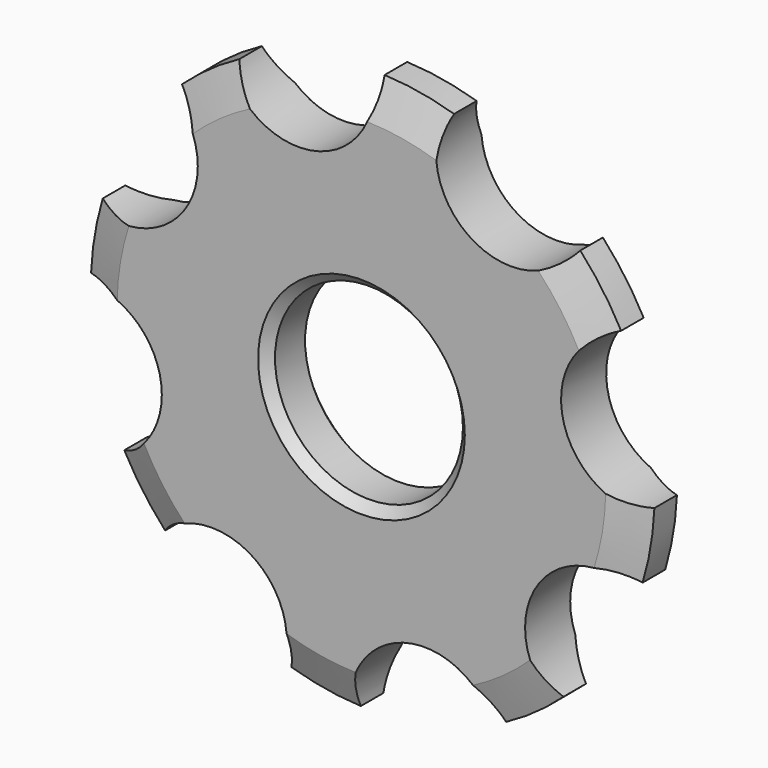
from build123d import *

# Parameters (mm, degrees)
F0_R         = 5
F1_DEPTH     = 3
F2_C1_SIZE2  = 0.75
F2_C1_SIZE   = 2
F2_C2_SIZE2  = 0.75
F2_C2_SIZE   = 2
F2_C3_SIZE2  = 0.75
F2_C3_SIZE   = 2
F2_C4_SIZE2  = 0.75
F2_C4_SIZE   = 2
F2_C5_SIZE2  = 0.75
F2_C5_SIZE   = 2
F2_C6_SIZE2  = 0.75
F2_C6_SIZE   = 2
F2_C7_SIZE2  = 0.75
F2_C7_SIZE   = 2
F2_C8_SIZE2  = 0.75
F2_C8_SIZE   = 2
F2_C9_SIZE2  = 2
F2_C9_SIZE   = 0.75
F2_C10_SIZE2 = 0.75
F2_C10_SIZE  = 2
F2_C11_SIZE2 = 0.75
F2_C11_SIZE  = 2
F2_C12_SIZE2 = 0.75
F2_C12_SIZE  = 2
F2_C13_SIZE2 = 0.75
F2_C13_SIZE  = 2
F2_C14_SIZE2 = 0.75
F2_C14_SIZE  = 2
F2_C15_SIZE2 = 0.75
F2_C15_SIZE  = 2
F2_C16_SIZE2 = 0.75
F2_C16_SIZE  = 2
F4_SIZE      = 0.5


# Not quite as in the source:
# - two fillets or chamfers of one size are made in one step


with BuildPart() as f1:
    # F0 (on Front) → F1 (new body)
    with BuildSketch(Plane.XZ):
        with BuildLine():
            ThreePointArc((14.98661002, -0.6336561441), (10.7222272749, 2.4563880526), (13.2160968729, 7.0947010823))
            ThreePointArc((13.2160968729, 7.0947010823), (12.2264008787, 8.6899437025), (11.0451961285, 10.1490710157))
            ThreePointArc((11.0451961285, 10.1490710157), (5.8448309663, 9.3186882647), (4.3284804738, 14.3619029654))
            ThreePointArc((4.3284804738, 14.3619029654), (2.5006528507, 14.790089091), (0.6336561441, 14.98661002))
            ThreePointArc((0.6336561441, 14.98661002), (0.6461967949, 14.8041057756), (0.6503799283, 14.6212190113))
            ThreePointArc((0.6503799283, 14.6212190113), (-2.6355906754, 10.6854646971), (-7.0947010823, 13.2160968729))
            ThreePointArc((-7.0947010823, 13.2160968729), (-8.6899437025, 12.2264008787), (-10.1490710157, 11.0451961285))
            ThreePointArc((-10.1490710157, 11.0451961285), (-9.0856364951, 9.6683222969), (-8.7073021792, 7.970224045))
            ThreePointArc((-8.7073021792, 7.970224045), (-10.5414770644, 4.6073084094), (-14.3619029654, 4.3284804738))
            ThreePointArc((-14.3619029654, 4.3284804738), (-14.790089091, 2.5006528507), (-14.98661002, 0.6336561441))
            ThreePointArc((-14.98661002, 0.6336561441), (-11.9250702797, -0.3948303977), (-10.6212190113, -3.3496200717))
            ThreePointArc((-10.6212190113, -3.3496200717), (-11.3333254186, -5.6277236082), (-13.2160968729, -7.0947010823))
            ThreePointArc((-13.2160968729, -7.0947010823), (-12.2264008787, -8.6899437025), (-11.0451961285, -10.1490710157))
            ThreePointArc((-11.0451961285, -10.1490710157), (-6.6100564697, -8.9456610257), (-3.970224045, -12.7073021792))
            ThreePointArc((-3.970224045, -12.7073021792), (-4.060813969, -13.5537730042), (-4.3284804738, -14.3619029654))
            ThreePointArc((-4.3284804738, -14.3619029654), (-2.5006528507, -14.790089091), (-0.6336561441, -14.98661002))
            ThreePointArc((-0.6336561441, -14.98661002), (2.4563880526, -10.7222272749), (7.0947010823, -13.2160968729))
            ThreePointArc((7.0947010823, -13.2160968729), (8.6899437025, -12.2264008787), (10.1490710157, -11.0451961285))
            ThreePointArc((10.1490710157, -11.0451961285), (9.3186882647, -5.8448309663), (14.3619029654, -4.3284804738))
            ThreePointArc((14.3619029654, -4.3284804738), (14.790089091, -2.5006528507), (14.98661002, -0.6336561441))
        make_face()
        Circle(F0_R, mode=Mode.SUBTRACT)
    extrude(amount=F1_DEPTH)

    # F2: chamfer of 2 x 0.75 on 16 edges, made by hand

    # F2_c1
    f2_c1_edges = [f1.edges().sort_by_distance(p)[0] for p in [
        (8.6899437025, -3, -12.2264008787),
    ]]
    f2_c1_side = f1.faces().sort_by_distance((8.6812537588, -3, -12.2141744779))[0]
    chamfer(f2_c1_edges, length=F2_C1_SIZE, length2=F2_C1_SIZE2, reference=f2_c1_side)

    # F2_c2
    f2_c2_edges = [f1.edges().sort_by_distance(p)[0] for p in [
        (14.790089091, -3, -2.5006528507),
    ]]
    f2_c2_side = f1.faces().sort_by_distance((14.7752990019, -3, -2.4981521978))[0]
    chamfer(f2_c2_edges, length=F2_C2_SIZE, length2=F2_C2_SIZE2, reference=f2_c2_side)

    # F2_c3
    f2_c3_edges = [f1.edges().sort_by_distance(p)[0] for p in [
        (12.2264008787, -3, 8.6899437025),
    ]]
    f2_c3_side = f1.faces().sort_by_distance((12.2141744779, -3, 8.6812537588))[0]
    chamfer(f2_c3_edges, length=F2_C3_SIZE, length2=F2_C3_SIZE2, reference=f2_c3_side)

    # F2_c4
    f2_c4_edges = [f1.edges().sort_by_distance(p)[0] for p in [
        (2.5006528507, -3, 14.790089091),
    ]]
    f2_c4_side = f1.faces().sort_by_distance((2.4981521978, -3, 14.7752990019))[0]
    chamfer(f2_c4_edges, length=F2_C4_SIZE, length2=F2_C4_SIZE2, reference=f2_c4_side)

    # F2_c5
    f2_c5_edges = [f1.edges().sort_by_distance(p)[0] for p in [
        (-8.6899437025, -3, 12.2264008787),
    ]]
    f2_c5_side = f1.faces().sort_by_distance((-8.6812537588, -3, 12.2141744779))[0]
    chamfer(f2_c5_edges, length=F2_C5_SIZE, length2=F2_C5_SIZE2, reference=f2_c5_side)

    # F2_c6
    f2_c6_edges = [f1.edges().sort_by_distance(p)[0] for p in [
        (-14.790089091, -3, 2.5006528507),
    ]]
    f2_c6_side = f1.faces().sort_by_distance((-14.7752990019, -3, 2.4981521978))[0]
    chamfer(f2_c6_edges, length=F2_C6_SIZE, length2=F2_C6_SIZE2, reference=f2_c6_side)

    # F2_c7
    f2_c7_edges = [f1.edges().sort_by_distance(p)[0] for p in [
        (-12.2264008787, -3, -8.6899437025),
    ]]
    f2_c7_side = f1.faces().sort_by_distance((-12.2141744779, -3, -8.6812537588))[0]
    chamfer(f2_c7_edges, length=F2_C7_SIZE, length2=F2_C7_SIZE2, reference=f2_c7_side)

    # F2_c8
    f2_c8_edges = [f1.edges().sort_by_distance(p)[0] for p in [
        (-2.5006528507, -3, -14.790089091),
    ]]
    f2_c8_side = f1.faces().sort_by_distance((-2.4981521978, -3, -14.7752990019))[0]
    chamfer(f2_c8_edges, length=F2_C8_SIZE, length2=F2_C8_SIZE2, reference=f2_c8_side)

    # F2_c9
    f2_c9_edges = [f1.edges().sort_by_distance(p)[0] for p in [
        (-12.2264008787, 0, -8.6899437025),
    ]]
    f2_c9_side = f1.faces().sort_by_distance((-12.2264008787, -0.015, -8.6899437025))[0]
    chamfer(f2_c9_edges, length=F2_C9_SIZE, length2=F2_C9_SIZE2, reference=f2_c9_side)

    # F2_c10
    f2_c10_edges = [f1.edges().sort_by_distance(p)[0] for p in [
        (-14.790089091, 0, 2.5006528507),
    ]]
    f2_c10_side = f1.faces().sort_by_distance((-14.7752990019, 0, 2.4981521978))[0]
    chamfer(f2_c10_edges, length=F2_C10_SIZE, length2=F2_C10_SIZE2, reference=f2_c10_side)

    # F2_c11
    f2_c11_edges = [f1.edges().sort_by_distance(p)[0] for p in [
        (-8.6899437025, 0, 12.2264008787),
    ]]
    f2_c11_side = f1.faces().sort_by_distance((-8.6812537588, 0, 12.2141744779))[0]
    chamfer(f2_c11_edges, length=F2_C11_SIZE, length2=F2_C11_SIZE2, reference=f2_c11_side)

    # F2_c12
    f2_c12_edges = [f1.edges().sort_by_distance(p)[0] for p in [
        (2.5006528507, 0, 14.790089091),
    ]]
    f2_c12_side = f1.faces().sort_by_distance((2.4981521978, 0, 14.7752990019))[0]
    chamfer(f2_c12_edges, length=F2_C12_SIZE, length2=F2_C12_SIZE2, reference=f2_c12_side)

    # F2_c13
    f2_c13_edges = [f1.edges().sort_by_distance(p)[0] for p in [
        (12.2264008787, 0, 8.6899437025),
    ]]
    f2_c13_side = f1.faces().sort_by_distance((12.2141744779, 0, 8.6812537588))[0]
    chamfer(f2_c13_edges, length=F2_C13_SIZE, length2=F2_C13_SIZE2, reference=f2_c13_side)

    # F2_c14
    f2_c14_edges = [f1.edges().sort_by_distance(p)[0] for p in [
        (14.790089091, 0, -2.5006528507),
    ]]
    f2_c14_side = f1.faces().sort_by_distance((14.7752990019, 0, -2.4981521978))[0]
    chamfer(f2_c14_edges, length=F2_C14_SIZE, length2=F2_C14_SIZE2, reference=f2_c14_side)

    # F2_c15
    f2_c15_edges = [f1.edges().sort_by_distance(p)[0] for p in [
        (8.6899437025, 0, -12.2264008787),
    ]]
    f2_c15_side = f1.faces().sort_by_distance((8.6812537588, 0, -12.2141744779))[0]
    chamfer(f2_c15_edges, length=F2_C15_SIZE, length2=F2_C15_SIZE2, reference=f2_c15_side)

    # F2_c16
    f2_c16_edges = [f1.edges().sort_by_distance(p)[0] for p in [
        (-2.5006528507, 0, -14.790089091),
    ]]
    f2_c16_side = f1.faces().sort_by_distance((-2.4981521978, 0, -14.7752990019))[0]
    chamfer(f2_c16_edges, length=F2_C16_SIZE, length2=F2_C16_SIZE2, reference=f2_c16_side)

    # F4
    f4_edges = [f1.edges().sort_by_distance(p)[0] for p in [
        (-5, -3, 0),
        (-5, 0, 0),
    ]]
    chamfer(f4_edges, length=F4_SIZE)


solid = f1.part
